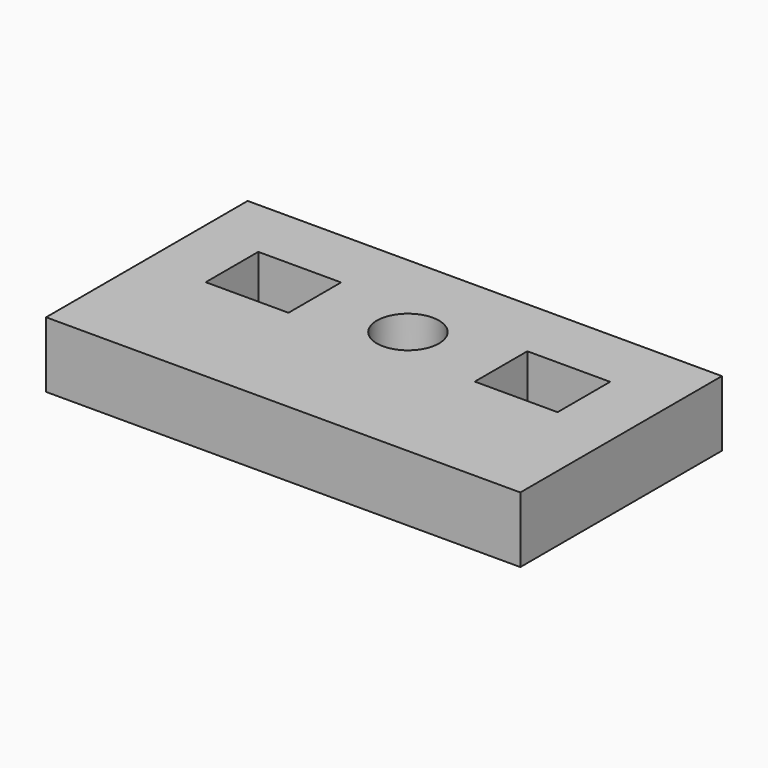
from build123d import *

# Parameters (mm, degrees)
F0_W     = 22.9125
F0_H     = 12.175
F0_W_2   = 4
F0_H_2   = 3.175
F0_R     = 1.5
F1_DEPTH = 3.175


# Not quite as in the source:
# - a length typed as a fraction of an inch, garbled in the dataset ("3 / 203.2 mm" for 3/8 in), is restored


with BuildPart() as f1:
    # F0 (on Top) → F1 (new body)
    with BuildSketch(Plane.XY):
        with Locations((-5.7368283796, -28.2098180865)):
            Rectangle(F0_W, F0_H)
        with Locations((-12.2805783796, -26.7098180865)):
            Rectangle(F0_W_2, F0_H_2, mode=Mode.SUBTRACT)
        with Locations((-5.7805783796, -26.7098180865)):
            Circle(F0_R, mode=Mode.SUBTRACT)
        with Locations((0.7194216204, -26.7098180865)):
            Rectangle(F0_W_2, F0_H_2, mode=Mode.SUBTRACT)
    extrude(amount=F1_DEPTH)


solid = f1.part
